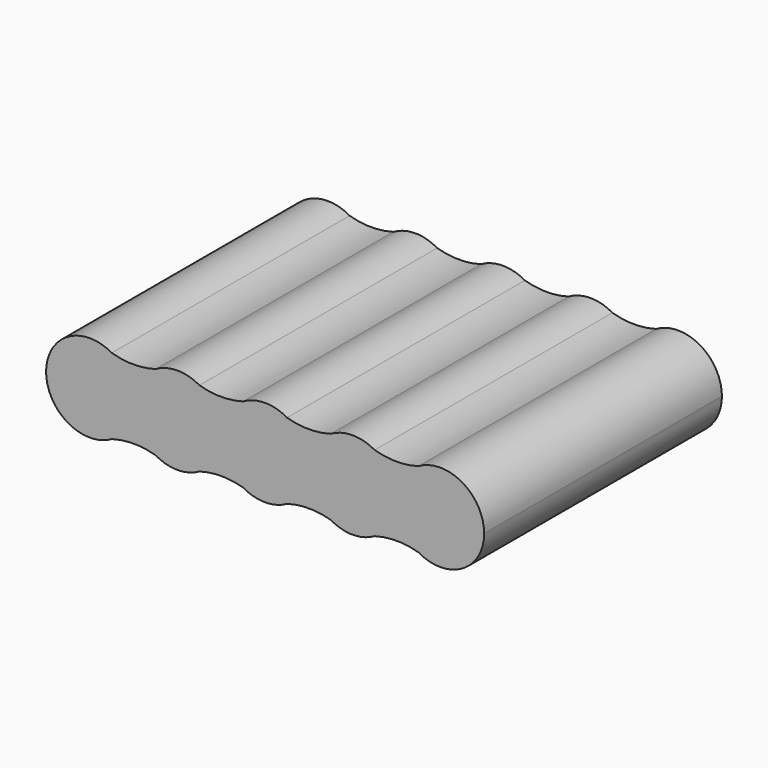
from build123d import *

# Parameters (mm, degrees)
F1_DEPTH = 48.26


# Not quite as in the source:
# - a feature names something its author has since deleted; it is built from what else it names


with BuildPart() as f1:
    # F0 (on Front) → F1 (new body)
    with BuildSketch(Plane.XZ):
        with BuildLine():
            ThreePointArc((3.556, -6.1591726717), (6.1591726717, -3.556), (7.112, 0))
            ThreePointArc((7.112, 0), (6.1591726717, 3.556), (3.556, 6.1591726717))
            ThreePointArc((3.556, 6.1591726717), (0, 7.112), (-3.556, 6.1591726717))
            ThreePointArc((-3.556, 6.1591726717), (-6.1591726717, 3.556), (-7.112, 0))
            ThreePointArc((-7.112, 0), (-6.1591726717, -3.556), (-3.556, -6.1591726717))
            ThreePointArc((-3.556, -6.1591726717), (0, -7.112), (3.556, -6.1591726717))
        make_face()
        with BuildLine():
            ThreePointArc((-10.668, -6.1591726717), (-8.0648273283, -3.556), (-7.112, 0))
            ThreePointArc((-7.112, 0), (-8.0648273283, 3.556), (-10.668, 6.1591726717))
            ThreePointArc((-10.668, 6.1591726717), (-14.224, 7.112), (-17.78, 6.1591726717))
            ThreePointArc((-17.78, 6.1591726717), (-20.3831726717, 3.556), (-21.336, 0))
            ThreePointArc((-21.336, 0), (-20.3831726717, -3.556), (-17.78, -6.1591726717))
            ThreePointArc((-17.78, -6.1591726717), (-14.224, -7.112), (-10.668, -6.1591726717))
        make_face()
        with BuildLine():
            ThreePointArc((-24.892, -6.1591726717), (-22.2888273283, -3.556), (-21.336, 0))
            ThreePointArc((-21.336, 0), (-22.2888273283, 3.556), (-24.892, 6.1591726717))
            ThreePointArc((-24.892, 6.1591726717), (-35.56, 0), (-24.892, -6.1591726717))
        make_face()
        with BuildLine():
            ThreePointArc((10.668, 6.1591726717), (8.0648273283, 3.556), (7.112, 0))
            ThreePointArc((7.112, 0), (8.0648273283, -3.556), (10.668, -6.1591726717))
            ThreePointArc((10.668, -6.1591726717), (14.224, -7.112), (17.78, -6.1591726717))
            ThreePointArc((17.78, -6.1591726717), (20.3831726717, -3.556), (21.336, 0))
            ThreePointArc((21.336, 0), (20.3831726717, 3.556), (17.78, 6.1591726717))
            ThreePointArc((17.78, 6.1591726717), (14.224, 7.112), (10.668, 6.1591726717))
        make_face()
        with BuildLine():
            ThreePointArc((24.892, 6.1591726717), (22.2888273283, 3.556), (21.336, 0))
            ThreePointArc((21.336, 0), (22.2888273283, -3.556), (24.892, -6.1591726717))
            ThreePointArc((24.892, -6.1591726717), (32.004, -6.1591726717), (35.56, 0))
            ThreePointArc((35.56, 0), (32.004, 6.1591726717), (24.892, 6.1591726717))
        make_face()
        with BuildLine():
            ThreePointArc((3.556, 6.1591726717), (6.1591726717, 3.556), (7.112, 0))
            ThreePointArc((7.112, 0), (8.0648273283, 3.556), (10.668, 6.1591726717))
            ThreePointArc((10.668, 6.1591726717), (7.112, 5.6520452644), (3.556, 6.1591726717))
        make_face()
        with BuildLine():
            ThreePointArc((24.892, 6.1591726717), (21.336, 5.6520452644), (17.78, 6.1591726717))
            ThreePointArc((17.78, 6.1591726717), (20.3831726717, 3.556), (21.336, 0))
            ThreePointArc((21.336, 0), (22.2888273283, 3.556), (24.892, 6.1591726717))
        make_face()
        with BuildLine():
            ThreePointArc((-7.112, 0), (-6.1591726717, 3.556), (-3.556, 6.1591726717))
            ThreePointArc((-3.556, 6.1591726717), (-7.112, 5.6520452644), (-10.668, 6.1591726717))
            ThreePointArc((-10.668, 6.1591726717), (-8.0648273283, 3.556), (-7.112, 0))
        make_face()
        with BuildLine():
            ThreePointArc((-21.336, 0), (-20.3831726717, 3.556), (-17.78, 6.1591726717))
            ThreePointArc((-17.78, 6.1591726717), (-21.336, 5.6520452644), (-24.892, 6.1591726717))
            ThreePointArc((-24.892, 6.1591726717), (-22.2888273283, 3.556), (-21.336, 0))
        make_face()
        with BuildLine():
            ThreePointArc((-24.892, -6.1591726717), (-21.336, -5.6520452644), (-17.78, -6.1591726717))
            ThreePointArc((-17.78, -6.1591726717), (-20.3831726717, -3.556), (-21.336, 0))
            ThreePointArc((-21.336, 0), (-22.2888273283, -3.556), (-24.892, -6.1591726717))
        make_face()
        with BuildLine():
            ThreePointArc((-10.668, -6.1591726717), (-7.112, -5.6520452644), (-3.556, -6.1591726717))
            ThreePointArc((-3.556, -6.1591726717), (-6.1591726717, -3.556), (-7.112, 0))
            ThreePointArc((-7.112, 0), (-8.0648273283, -3.556), (-10.668, -6.1591726717))
        make_face()
        with BuildLine():
            ThreePointArc((10.668, -6.1591726717), (8.0648273283, -3.556), (7.112, 0))
            ThreePointArc((7.112, 0), (6.1591726717, -3.556), (3.556, -6.1591726717))
            ThreePointArc((3.556, -6.1591726717), (7.112, -5.6520452644), (10.668, -6.1591726717))
        make_face()
        with BuildLine():
            ThreePointArc((21.336, 0), (20.3831726717, -3.556), (17.78, -6.1591726717))
            ThreePointArc((17.78, -6.1591726717), (21.336, -5.6520452644), (24.892, -6.1591726717))
            ThreePointArc((24.892, -6.1591726717), (22.2888273283, -3.556), (21.336, 0))
        make_face()
    extrude(amount=F1_DEPTH)


solid = f1.part
